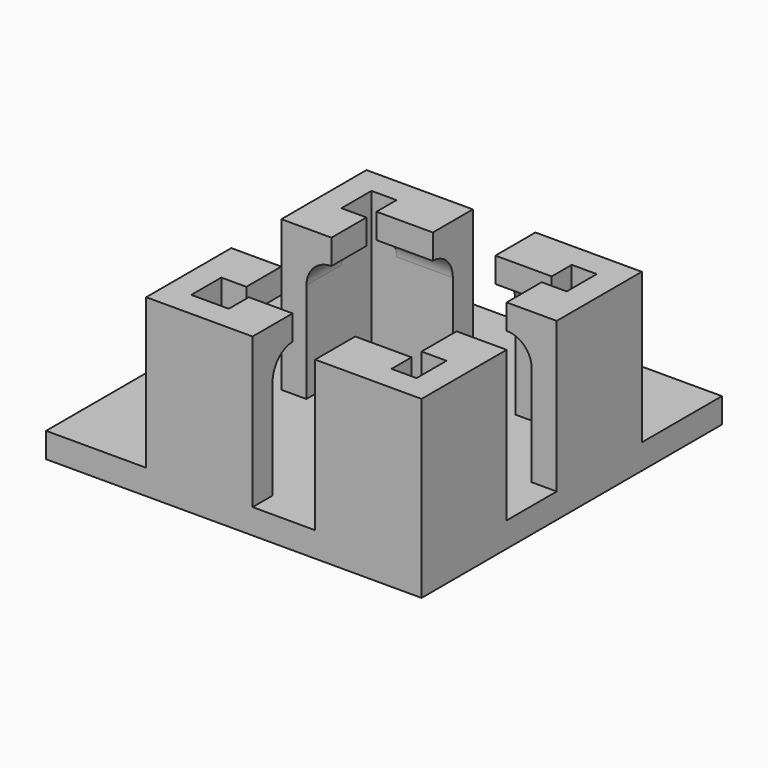
from build123d import *

# Parameters (mm, degrees)
F0_W     = 30
F0_H     = 30
F1_DEPTH = 2
F2_W     = 22
F2_H     = 22
F2_W_2   = 18
F2_H_2   = 18
F3_DEPTH = 10
F4_W     = 22
F4_H     = 22
F4_W_2   = 2
F4_H_2   = 12
F4_W_3   = 14
F4_H_3   = 2
F4_W_4   = 13
F5_DEPTH = 2
F6_R     = 1.99999
F7_W     = 12.5
F7_H     = 5
F7_W_2   = 5
F7_H_2   = 12.5
F8_DEPTH = 12


# Not quite as in the source:
# - a fillet or chamfer is up to 0.001 mm smaller than in the source, because OpenCascade refuses the exact size


with BuildPart() as f1:
    # F0 (on Top) → F1 (new body)
    with BuildSketch(Plane.XY):
        with Locations((15, -15)):
            Rectangle(F0_W, F0_H)
    extrude(amount=F1_DEPTH)

    # F2 (on face) → F3 (join)
    with BuildSketch(Plane.XY.offset(2)):
        with Locations((19, -19)):
            Rectangle(F2_W, F2_H)
        with Locations((19, -19)):
            Rectangle(F2_W_2, F2_H_2, mode=Mode.SUBTRACT)
    extrude(amount=F3_DEPTH)

    # F4 (on face) → F5 (join)
    with BuildSketch(Plane.XY.offset(12)):
        with Locations((19, -19)):
            Rectangle(F4_W, F4_H)
        Polygon((13, -28), (10, -28), (10, -25), (10, -13), (10, -10), (12, -10), (26, -10), (28, -10), (28, -13), (28, -25), (28, -28), (26, -28), align=None, mode=Mode.SUBTRACT)
        with Locations((11, -19)):
            Rectangle(F4_W_2, F4_H_2)
        with Locations((19, -11)):
            Rectangle(F4_W_3, F4_H_3)
        with Locations((27, -19)):
            Rectangle(F4_W_2, F4_H_2)
        with Locations((19.5, -27)):
            Rectangle(F4_W_4, F4_H_3)
    extrude(amount=F5_DEPTH)

    # F6 (radius 2 in the source; OpenCascade refuses exactly that, so slightly less here)
    f6_edges = [f1.edges().sort_by_distance(p)[0] for p in [
        (10, -19, 12),
        (28, -19, 12),
        (19, -10, 12),
        (19.5, -28, 12),
    ]]
    fillet(f6_edges, radius=F6_R)

    # F7 (on face) → F8 (cut, through all)
    with BuildSketch(Plane.XY.offset(14)):
        with Locations((27.75, -19)):
            Rectangle(F7_W, F7_H)
        with Locations((19, -27.75)):
            Rectangle(F7_W_2, F7_H_2)
        with Locations((19, -19)):
            Rectangle(F7_W_2, F7_H)
        with Locations((10.25, -19)):
            Rectangle(F7_W, F7_H)
        with Locations((19, -10.25)):
            Rectangle(F7_W_2, F7_H_2)
    extrude(amount=-F8_DEPTH, mode=Mode.SUBTRACT)


solid = f1.part
